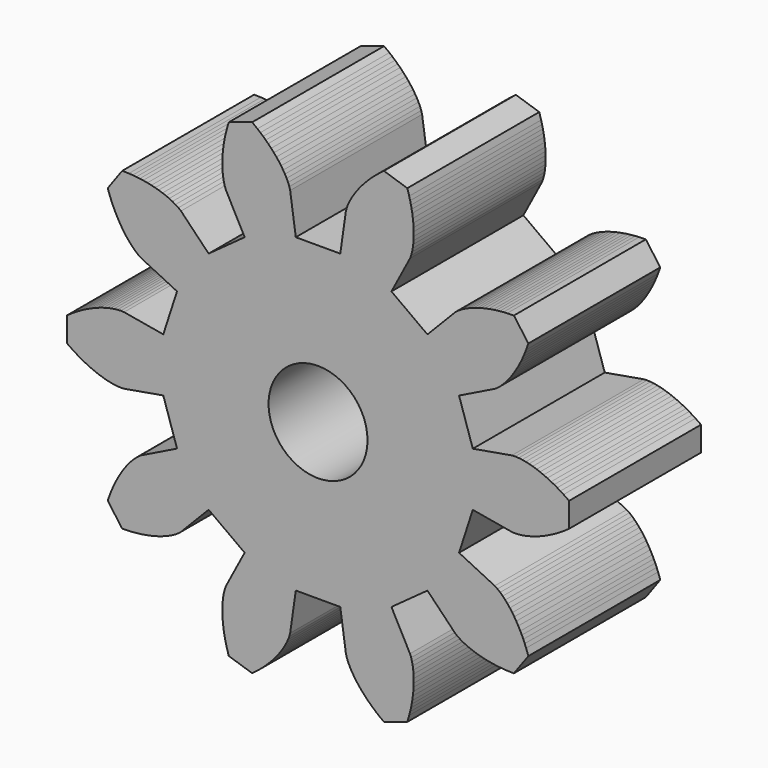
from build123d import *

# Parameters (mm, degrees)
F0_R     = 1.5
F1_DEPTH = 5


# Not quite as in the source:
# - ends of sketch curves that miss each other by under 0.0002 mm in the source are joined


with BuildPart() as f1:
    # F0 (on Front) → F1 (new body)
    with BuildSketch(Plane.XZ):
        with BuildLine():
            ThreePointArc((4.2753417889, -0.9237346066), (4.4837280553, -0.2822940953), (4.6921702972, 0.3591282284))
            Line((4.6921702972, 0.3591282284), (5.878934, 0.152889))
            Line((5.878934, 0.152889), (5.978914, 0.147897))
            Line((5.978914, 0.147897), (6.083031, 0.153397))
            Line((6.083031, 0.153397), (6.188792, 0.166293))
            Line((6.188792, 0.166293), (6.296123, 0.185564))
            Line((6.296123, 0.185564), (6.39688, 0.208667))
            Line((6.39688, 0.208667), (6.507485, 0.239158))
            Line((6.507485, 0.239158), (6.627466, 0.277934))
            Line((6.627466, 0.277934), (6.729844, 0.315505))
            Line((6.729844, 0.315505), (6.837582, 0.359366))
            Line((6.837582, 0.359366), (6.95036, 0.409935))
            Line((6.95036, 0.409935), (7.067828, 0.467611))
            Line((7.067828, 0.467611), (7.158791, 0.515766))
            Line((7.158791, 0.515766), (7.252025, 0.568292))
            Line((7.252025, 0.568292), (7.347362, 0.62534))
            Line((7.347362, 0.62534), (7.444626, 0.687056))
            Line((7.444626, 0.687056), (7.610854, 0.801339))
            Line((7.610854, 0.801339), (7.610854, 1.547781))
            Line((7.610854, 1.547781), (7.444624, 1.662064))
            Line((7.444624, 1.662064), (7.347361, 1.723779))
            Line((7.347361, 1.723779), (7.252025, 1.780827))
            Line((7.252025, 1.780827), (7.15879, 1.833354))
            Line((7.15879, 1.833354), (7.067828, 1.881508))
            Line((7.067828, 1.881508), (6.950358, 1.939185))
            Line((6.950358, 1.939185), (6.837582, 1.989753))
            Line((6.837582, 1.989753), (6.729843, 2.033614))
            Line((6.729843, 2.033614), (6.627464, 2.071186))
            Line((6.627464, 2.071186), (6.507485, 2.109962))
            Line((6.507485, 2.109962), (6.39688, 2.140452))
            Line((6.39688, 2.140452), (6.296123, 2.163555))
            Line((6.296123, 2.163555), (6.188792, 2.182826))
            Line((6.188792, 2.182826), (6.08303, 2.195722))
            Line((6.08303, 2.195722), (5.978914, 2.201222))
            Line((5.978914, 2.201222), (5.878933, 2.19623))
            Line((5.878933, 2.19623), (4.692172, 1.989989))
            ThreePointArc((4.692172, 1.989989), (4.4837309325, 2.6314120428), (4.2753451638, 3.2728530532))
            Line((4.2753451638, 3.2728530532), (5.35668, 3.80356))
            Line((5.35668, 3.80356), (5.4405, 3.858289))
            Line((5.4405, 3.858289), (5.5215, 3.923937))
            Line((5.5215, 3.923937), (5.599482, 3.996535))
            Line((5.599482, 3.996535), (5.674988, 4.075213))
            Line((5.674988, 4.075213), (5.742922, 4.153126))
            Line((5.742922, 4.153126), (5.814482, 4.242806))
            Line((5.814482, 4.242806), (5.888756, 4.344699))
            Line((5.888756, 4.344699), (5.949498, 4.435272))
            Line((5.949498, 4.435272), (6.010879, 4.534083))
            Line((6.010879, 4.534083), (6.072394, 4.641282))
            Line((6.072394, 4.641282), (6.133527, 4.75699))
            Line((6.133527, 4.75699), (6.178813, 4.849415))
            Line((6.178813, 4.849415), (6.223367, 4.946711))
            Line((6.223367, 4.946711), (6.266963, 5.048901))
            Line((6.266963, 5.048901), (6.309377, 5.156001))
            Line((6.309377, 5.156001), (6.376684, 5.346164))
            Line((6.376684, 5.346164), (5.937936, 5.950048))
            Line((5.937936, 5.950048), (5.73628, 5.944798))
            Line((5.73628, 5.944798), (5.621317, 5.937556))
            Line((5.621317, 5.937556), (5.510656, 5.927672))
            Line((5.510656, 5.927672), (5.404354, 5.915365))
            Line((5.404354, 5.915365), (5.302459, 5.900857))
            Line((5.302459, 5.900857), (5.173523, 5.878471))
            Line((5.173523, 5.878471), (5.052562, 5.853093))
            Line((5.052562, 5.853093), (4.939618, 5.825251))
            Line((4.939618, 5.825251), (4.834708, 5.79547))
            Line((4.834708, 5.79547), (4.714851, 5.756318))
            Line((4.714851, 5.756318), (4.607447, 5.715973))
            Line((4.607447, 5.715973), (4.512354, 5.67544))
            Line((4.512354, 5.67544), (4.414194, 5.627943))
            Line((4.414194, 5.627943), (4.321051, 5.576212))
            Line((4.321051, 5.576212), (4.233586, 5.519463))
            Line((4.233586, 5.519463), (4.155634, 5.456658))
            Line((4.155634, 5.456658), (3.31675, 4.592245))
            ThreePointArc((3.31675, 4.592245), (2.7710979645, 4.9886473644), (2.2254808469, 5.3850977893))
            Line((2.2254808469, 5.3850977893), (2.788358, 6.450042))
            Line((2.788358, 6.450042), (2.824001, 6.543587))
            Line((2.824001, 6.543587), (2.850944, 6.644307))
            Line((2.850944, 6.644307), (2.871361, 6.748877))
            Line((2.871361, 6.748877), (2.886201, 6.856911))
            Line((2.886201, 6.856911), (2.895364, 6.959874))
            Line((2.895364, 6.959874), (2.900545, 7.074489))
            Line((2.900545, 7.074489), (2.900742, 7.200579))
            Line((2.900742, 7.200579), (2.896647, 7.309556))
            Line((2.896647, 7.309556), (2.888225, 7.425575))
            Line((2.888225, 7.425575), (2.874982, 7.548459))
            Line((2.874982, 7.548459), (2.856428, 7.678002))
            Line((2.856428, 7.678002), (2.83874, 7.779394))
            Line((2.83874, 7.779394), (2.817595, 7.884296))
            Line((2.817595, 7.884296), (2.792799, 7.992596))
            Line((2.792799, 7.992596), (2.76416, 8.10417))
            Line((2.76416, 8.10417), (2.706839, 8.297578))
            Line((2.706839, 8.297578), (1.99693, 8.528241))
            Line((1.99693, 8.528241), (1.836873, 8.405463))
            Line((1.836873, 8.405463), (1.748122, 8.332031))
            Line((1.748122, 8.332031), (1.664405, 8.258989))
            Line((1.664405, 8.258989), (1.585639, 8.186549))
            Line((1.585639, 8.186549), (1.511732, 8.11492))
            Line((1.511732, 8.11492), (1.420578, 8.021022))
            Line((1.420578, 8.021022), (1.337635, 7.929392))
            Line((1.337635, 7.929392), (1.262627, 7.840481))
            Line((1.262627, 7.840481), (1.195258, 7.754723))
            Line((1.195258, 7.754723), (1.121305, 7.652599))
            Line((1.121305, 7.652599), (1.058128, 7.556829))
            Line((1.058128, 7.556829), (1.00502, 7.468143))
            Line((1.00502, 7.468143), (0.953525, 7.37202))
            Line((0.953525, 7.37202), (0.908577, 7.27542))
            Line((0.908577, 7.27542), (0.871173, 7.178099))
            Line((0.871173, 7.178099), (0.845025, 7.081469))
            Line((0.845025, 7.081469), (0.674443, 5.88906))
            ThreePointArc((0.674443, 5.88906), (1.5e-06, 5.8890320012), (-0.67444, 5.8890618078))
            Line((-0.67444, 5.8890618078), (-0.845022, 7.08147))
            Line((-0.845022, 7.08147), (-0.87117, 7.178099))
            Line((-0.87117, 7.178099), (-0.908574, 7.27542))
            Line((-0.908574, 7.27542), (-0.953521, 7.37202))
            Line((-0.953521, 7.37202), (-1.005016, 7.468143))
            Line((-1.005016, 7.468143), (-1.058124, 7.556829))
            Line((-1.058124, 7.556829), (-1.121301, 7.652598))
            Line((-1.121301, 7.652598), (-1.195255, 7.754725))
            Line((-1.195255, 7.754725), (-1.262624, 7.840481))
            Line((-1.262624, 7.840481), (-1.337632, 7.929392))
            Line((-1.337632, 7.929392), (-1.420575, 8.021024))
            Line((-1.420575, 8.021024), (-1.511728, 8.11492))
            Line((-1.511728, 8.11492), (-1.585636, 8.186551))
            Line((-1.585636, 8.186551), (-1.664402, 8.25899))
            Line((-1.664402, 8.25899), (-1.748119, 8.332032))
            Line((-1.748119, 8.332032), (-1.83687, 8.405464))
            Line((-1.83687, 8.405464), (-1.996926, 8.528241))
            Line((-1.996926, 8.528241), (-2.706835, 8.297578))
            Line((-2.706835, 8.297578), (-2.764157, 8.104169))
            Line((-2.764157, 8.104169), (-2.792795, 7.992595))
            Line((-2.792795, 7.992595), (-2.817591, 7.884296))
            Line((-2.817591, 7.884296), (-2.838736, 7.779392))
            Line((-2.838736, 7.779392), (-2.856425, 7.678002))
            Line((-2.856425, 7.678002), (-2.874978, 7.548459))
            Line((-2.874978, 7.548459), (-2.888221, 7.425576))
            Line((-2.888221, 7.425576), (-2.896643, 7.309556))
            Line((-2.896643, 7.309556), (-2.900739, 7.200578))
            Line((-2.900739, 7.200578), (-2.900542, 7.074489))
            Line((-2.900542, 7.074489), (-2.895361, 6.959875))
            Line((-2.895361, 6.959875), (-2.886197, 6.856911))
            Line((-2.886197, 6.856911), (-2.871358, 6.748877))
            Line((-2.871358, 6.748877), (-2.850941, 6.644307))
            Line((-2.850941, 6.644307), (-2.823998, 6.543587))
            Line((-2.823998, 6.543587), (-2.788355, 6.450042))
            Line((-2.788355, 6.450042), (-2.225478, 5.385097))
            ThreePointArc((-2.225478, 5.385097), (-2.771095971, 4.9886482498), (-3.3167477562, 4.592246041))
            Line((-3.3167477562, 4.592246041), (-4.155632, 5.456658))
            Line((-4.155632, 5.456658), (-4.233584, 5.519464))
            Line((-4.233584, 5.519464), (-4.321049, 5.576213))
            Line((-4.321049, 5.576213), (-4.414192, 5.627944))
            Line((-4.414192, 5.627944), (-4.512352, 5.675442))
            Line((-4.512352, 5.675442), (-4.607445, 5.715974))
            Line((-4.607445, 5.715974), (-4.714848, 5.756319))
            Line((-4.714848, 5.756319), (-4.834706, 5.795471))
            Line((-4.834706, 5.795471), (-4.939616, 5.825252))
            Line((-4.939616, 5.825252), (-5.052559, 5.853094))
            Line((-5.052559, 5.853094), (-5.173522, 5.878472))
            Line((-5.173522, 5.878472), (-5.302457, 5.900857))
            Line((-5.302457, 5.900857), (-5.404352, 5.915366))
            Line((-5.404352, 5.915366), (-5.510654, 5.927673))
            Line((-5.510654, 5.927673), (-5.621316, 5.937558))
            Line((-5.621316, 5.937558), (-5.736279, 5.944799))
            Line((-5.736279, 5.944799), (-5.937934, 5.950049))
            Line((-5.937934, 5.950049), (-6.376683, 5.346165))
            Line((-6.376683, 5.346165), (-6.309373, 5.156001))
            Line((-6.309373, 5.156001), (-6.266961, 5.048902))
            Line((-6.266961, 5.048902), (-6.223364, 4.946712))
            Line((-6.223364, 4.946712), (-6.17881, 4.849415))
            Line((-6.17881, 4.849415), (-6.133525, 4.756991))
            Line((-6.133525, 4.756991), (-6.072391, 4.641283))
            Line((-6.072391, 4.641283), (-6.010877, 4.534084))
            Line((-6.010877, 4.534084), (-5.949495, 4.435272))
            Line((-5.949495, 4.435272), (-5.888753, 4.344699))
            Line((-5.888753, 4.344699), (-5.81448, 4.242807))
            Line((-5.81448, 4.242807), (-5.74292, 4.153128))
            Line((-5.74292, 4.153128), (-5.674986, 4.075214))
            Line((-5.674986, 4.075214), (-5.59948, 3.996536))
            Line((-5.59948, 3.996536), (-5.521498, 3.923937))
            Line((-5.521498, 3.923937), (-5.440498, 3.85829))
            Line((-5.440498, 3.85829), (-5.356678, 3.803561))
            Line((-5.356678, 3.803561), (-4.275343, 3.272853))
            ThreePointArc((-4.275343, 3.272853), (-4.4837282639, 2.6314121631), (-4.6921703347, 1.9899897838))
            Line((-4.6921703347, 1.9899897838), (-5.878932, 2.196231))
            Line((-5.878932, 2.196231), (-5.978913, 2.201222))
            Line((-5.978913, 2.201222), (-6.08303, 2.195723))
            Line((-6.08303, 2.195723), (-6.188791, 2.182826))
            Line((-6.188791, 2.182826), (-6.296122, 2.163555))
            Line((-6.296122, 2.163555), (-6.396879, 2.140453))
            Line((-6.396879, 2.140453), (-6.507485, 2.109962))
            Line((-6.507485, 2.109962), (-6.627465, 2.071186))
            Line((-6.627465, 2.071186), (-6.729843, 2.033615))
            Line((-6.729843, 2.033615), (-6.837581, 1.989753))
            Line((-6.837581, 1.989753), (-6.950359, 1.939185))
            Line((-6.950359, 1.939185), (-7.067828, 1.881509))
            Line((-7.067828, 1.881509), (-7.158791, 1.833354))
            Line((-7.158791, 1.833354), (-7.252025, 1.780828))
            Line((-7.252025, 1.780828), (-7.347361, 1.723779))
            Line((-7.347361, 1.723779), (-7.444625, 1.662064))
            Line((-7.444625, 1.662064), (-7.610853, 1.547781))
            Line((-7.610853, 1.547781), (-7.610853, 0.801339))
            Line((-7.610853, 0.801339), (-7.444624, 0.687056))
            Line((-7.444624, 0.687056), (-7.34736, 0.625341))
            Line((-7.34736, 0.625341), (-7.252024, 0.568293))
            Line((-7.252024, 0.568293), (-7.158789, 0.515766))
            Line((-7.158789, 0.515766), (-7.067828, 0.467612))
            Line((-7.067828, 0.467612), (-6.950358, 0.409935))
            Line((-6.950358, 0.409935), (-6.837581, 0.359367))
            Line((-6.837581, 0.359367), (-6.729843, 0.315506))
            Line((-6.729843, 0.315506), (-6.627464, 0.277934))
            Line((-6.627464, 0.277934), (-6.507485, 0.239159))
            Line((-6.507485, 0.239159), (-6.396879, 0.208668))
            Line((-6.396879, 0.208668), (-6.296122, 0.185565))
            Line((-6.296122, 0.185565), (-6.18879, 0.166294))
            Line((-6.18879, 0.166294), (-6.083029, 0.153398))
            Line((-6.083029, 0.153398), (-5.978913, 0.147898))
            Line((-5.978913, 0.147898), (-5.878932, 0.15289))
            Line((-5.878932, 0.15289), (-4.692171, 0.359131))
            ThreePointArc((-4.692171, 0.359131), (-4.4837298858, -0.2822915276), (-4.2753442362, -0.9237320767))
            Line((-4.2753442362, -0.9237320767), (-5.356681, -1.45444))
            Line((-5.356681, -1.45444), (-5.440501, -1.509168))
            Line((-5.440501, -1.509168), (-5.5215, -1.574816))
            Line((-5.5215, -1.574816), (-5.599482, -1.647414))
            Line((-5.599482, -1.647414), (-5.674988, -1.726092))
            Line((-5.674988, -1.726092), (-5.742923, -1.804005))
            Line((-5.742923, -1.804005), (-5.814482, -1.893685))
            Line((-5.814482, -1.893685), (-5.888757, -1.995578))
            Line((-5.888757, -1.995578), (-5.949499, -2.08615))
            Line((-5.949499, -2.08615), (-6.010879, -2.184962))
            Line((-6.010879, -2.184962), (-6.072395, -2.292162))
            Line((-6.072395, -2.292162), (-6.133528, -2.407869))
            Line((-6.133528, -2.407869), (-6.178814, -2.500294))
            Line((-6.178814, -2.500294), (-6.223368, -2.59759))
            Line((-6.223368, -2.59759), (-6.266964, -2.69978))
            Line((-6.266964, -2.69978), (-6.309378, -2.80688))
            Line((-6.309378, -2.80688), (-6.376685, -2.997043))
            Line((-6.376685, -2.997043), (-5.937937, -3.600927))
            Line((-5.937937, -3.600927), (-5.736281, -3.595677))
            Line((-5.736281, -3.595677), (-5.621318, -3.588435))
            Line((-5.621318, -3.588435), (-5.510657, -3.578551))
            Line((-5.510657, -3.578551), (-5.404354, -3.566244))
            Line((-5.404354, -3.566244), (-5.30246, -3.551736))
            Line((-5.30246, -3.551736), (-5.173523, -3.52935))
            Line((-5.173523, -3.52935), (-5.052562, -3.503972))
            Line((-5.052562, -3.503972), (-4.939619, -3.47613))
            Line((-4.939619, -3.47613), (-4.834708, -3.446349))
            Line((-4.834708, -3.446349), (-4.714851, -3.407198))
            Line((-4.714851, -3.407198), (-4.607448, -3.366853))
            Line((-4.607448, -3.366853), (-4.512355, -3.32632))
            Line((-4.512355, -3.32632), (-4.414194, -3.278822))
            Line((-4.414194, -3.278822), (-4.321052, -3.227091))
            Line((-4.321052, -3.227091), (-4.233587, -3.170342))
            Line((-4.233587, -3.170342), (-4.155635, -3.107537))
            Line((-4.155635, -3.107537), (-3.31675, -2.243124))
            ThreePointArc((-3.31675, -2.243124), (-2.7710983472, -2.6395268912), (-2.2254812543, -3.0359773499))
            Line((-2.2254812543, -3.0359773499), (-2.788359, -4.100922))
            Line((-2.788359, -4.100922), (-2.824002, -4.194467))
            Line((-2.824002, -4.194467), (-2.850945, -4.295187))
            Line((-2.850945, -4.295187), (-2.871362, -4.399757))
            Line((-2.871362, -4.399757), (-2.886201, -4.50779))
            Line((-2.886201, -4.50779), (-2.895365, -4.610754))
            Line((-2.895365, -4.610754), (-2.900546, -4.725369))
            Line((-2.900546, -4.725369), (-2.900744, -4.851459))
            Line((-2.900744, -4.851459), (-2.896648, -4.960437))
            Line((-2.896648, -4.960437), (-2.888226, -5.076456))
            Line((-2.888226, -5.076456), (-2.874983, -5.19934))
            Line((-2.874983, -5.19934), (-2.856429, -5.328883))
            Line((-2.856429, -5.328883), (-2.838741, -5.430275))
            Line((-2.838741, -5.430275), (-2.817596, -5.535177))
            Line((-2.817596, -5.535177), (-2.7928, -5.643476))
            Line((-2.7928, -5.643476), (-2.764162, -5.75505))
            Line((-2.764162, -5.75505), (-2.70684, -5.948458))
            Line((-2.70684, -5.948458), (-1.996931, -6.179121))
            Line((-1.996931, -6.179121), (-1.836874, -6.056343))
            Line((-1.836874, -6.056343), (-1.748123, -5.982912))
            Line((-1.748123, -5.982912), (-1.664406, -5.90987))
            Line((-1.664406, -5.90987), (-1.585639, -5.83743))
            Line((-1.585639, -5.83743), (-1.511733, -5.765801))
            Line((-1.511733, -5.765801), (-1.420579, -5.671903))
            Line((-1.420579, -5.671903), (-1.337636, -5.580273))
            Line((-1.337636, -5.580273), (-1.262628, -5.491361))
            Line((-1.262628, -5.491361), (-1.195259, -5.405603))
            Line((-1.195259, -5.405603), (-1.121305, -5.303479))
            Line((-1.121305, -5.303479), (-1.058128, -5.207709))
            Line((-1.058128, -5.207709), (-1.00502, -5.119023))
            Line((-1.00502, -5.119023), (-0.953526, -5.0229))
            Line((-0.953526, -5.0229), (-0.908578, -4.9263))
            Line((-0.908578, -4.9263), (-0.871174, -4.828979))
            Line((-0.871174, -4.828979), (-0.845026, -4.73235))
            Line((-0.845026, -4.73235), (-0.674443, -3.539941))
            ThreePointArc((-0.674443, -3.539941), (-1.5e-06, -3.5399120003), (0.67444, -3.5399416176))
            Line((0.67444, -3.5399416176), (0.845021, -4.732351))
            Line((0.845021, -4.732351), (0.87117, -4.82898))
            Line((0.87117, -4.82898), (0.908574, -4.926302))
            Line((0.908574, -4.926302), (0.953521, -5.022901))
            Line((0.953521, -5.022901), (1.005016, -5.119024))
            Line((1.005016, -5.119024), (1.058123, -5.20771))
            Line((1.058123, -5.20771), (1.1213, -5.30348))
            Line((1.1213, -5.30348), (1.195254, -5.405606))
            Line((1.195254, -5.405606), (1.262623, -5.491364))
            Line((1.262623, -5.491364), (1.337631, -5.580275))
            Line((1.337631, -5.580275), (1.420574, -5.671906))
            Line((1.420574, -5.671906), (1.511728, -5.765803))
            Line((1.511728, -5.765803), (1.585635, -5.837433))
            Line((1.585635, -5.837433), (1.664401, -5.909872))
            Line((1.664401, -5.909872), (1.748118, -5.982913))
            Line((1.748118, -5.982913), (1.836869, -6.056346))
            Line((1.836869, -6.056346), (1.996925, -6.179123))
            Line((1.996925, -6.179123), (2.706834, -5.94846))
            Line((2.706834, -5.94846), (2.764156, -5.755051))
            Line((2.764156, -5.755051), (2.792795, -5.643476))
            Line((2.792795, -5.643476), (2.817591, -5.535178))
            Line((2.817591, -5.535178), (2.838735, -5.430275))
            Line((2.838735, -5.430275), (2.856424, -5.328885))
            Line((2.856424, -5.328885), (2.874977, -5.199341))
            Line((2.874977, -5.199341), (2.888221, -5.076458))
            Line((2.888221, -5.076458), (2.896643, -4.960438))
            Line((2.896643, -4.960438), (2.900738, -4.851459))
            Line((2.900738, -4.851459), (2.900541, -4.725371))
            Line((2.900541, -4.725371), (2.89536, -4.610756))
            Line((2.89536, -4.610756), (2.886197, -4.507792))
            Line((2.886197, -4.507792), (2.871357, -4.399759))
            Line((2.871357, -4.399759), (2.850941, -4.295188))
            Line((2.850941, -4.295188), (2.823998, -4.194468))
            Line((2.823998, -4.194468), (2.788354, -4.100924))
            Line((2.788354, -4.100924), (2.225479, -3.035979))
            ThreePointArc((2.225479, -3.035979), (2.7710963565, -2.6395289039), (3.3167481995, -2.2431262746))
            Line((3.3167481995, -2.2431262746), (4.155631, -3.10754))
            Line((4.155631, -3.10754), (4.233583, -3.170346))
            Line((4.233583, -3.170346), (4.321048, -3.227095))
            Line((4.321048, -3.227095), (4.41419, -3.278826))
            Line((4.41419, -3.278826), (4.51235, -3.326324))
            Line((4.51235, -3.326324), (4.607444, -3.366856))
            Line((4.607444, -3.366856), (4.714847, -3.407201))
            Line((4.714847, -3.407201), (4.834705, -3.446354))
            Line((4.834705, -3.446354), (4.939615, -3.476134))
            Line((4.939615, -3.476134), (5.052558, -3.503976))
            Line((5.052558, -3.503976), (5.17352, -3.529355))
            Line((5.17352, -3.529355), (5.302456, -3.55174))
            Line((5.302456, -3.55174), (5.404351, -3.566249))
            Line((5.404351, -3.566249), (5.510653, -3.578556))
            Line((5.510653, -3.578556), (5.621314, -3.58844))
            Line((5.621314, -3.58844), (5.736278, -3.595682))
            Line((5.736278, -3.595682), (5.937933, -3.600932))
            Line((5.937933, -3.600932), (6.376681, -2.997048))
            Line((6.376681, -2.997048), (6.309372, -2.806883))
            Line((6.309372, -2.806883), (6.26696, -2.699785))
            Line((6.26696, -2.699785), (6.223363, -2.597595))
            Line((6.223363, -2.597595), (6.178809, -2.500297))
            Line((6.178809, -2.500297), (6.133524, -2.407874))
            Line((6.133524, -2.407874), (6.07239, -2.292165))
            Line((6.07239, -2.292165), (6.010875, -2.184966))
            Line((6.010875, -2.184966), (5.949495, -2.086155))
            Line((5.949495, -2.086155), (5.888752, -1.995582))
            Line((5.888752, -1.995582), (5.814479, -1.89369))
            Line((5.814479, -1.89369), (5.742919, -1.80401))
            Line((5.742919, -1.80401), (5.674985, -1.726096))
            Line((5.674985, -1.726096), (5.599479, -1.647418))
            Line((5.599479, -1.647418), (5.521497, -1.574819))
            Line((5.521497, -1.574819), (5.440498, -1.509172))
            Line((5.440498, -1.509172), (5.356677, -1.454443))
            Line((5.356677, -1.454443), (4.2753417889, -0.9237346066))
        make_face()
        with Locations((1e-06, 1.17456)):
            Circle(F0_R, mode=Mode.SUBTRACT)
    extrude(amount=F1_DEPTH)


solid = f1.part
